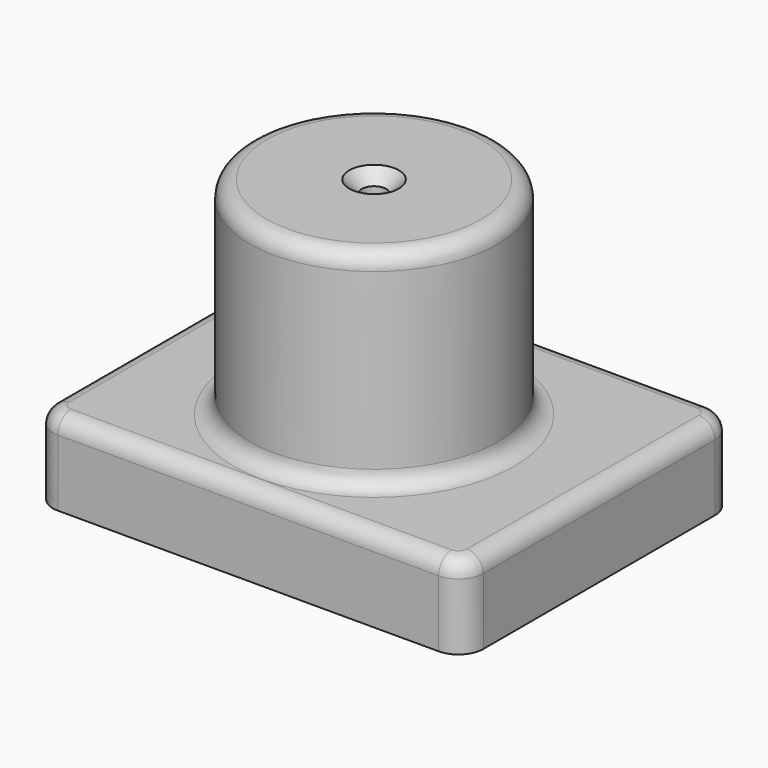
from build123d import *

# Parameters (mm, degrees)
F0_W            = 52
F0_H            = 41
F1_DEPTH        = 10
F3_DEPTH        = 20
F4_R            = 11
F5_DEPTH        = 10.001
F6_R            = 15
F7_DEPTH        = 5
F9_R            = 3
F10_R           = 11.5
F10_R_2         = 9.5
F11_DEPTH       = 35
F12_T3_DEPTH    = 35
F12_T5_DEPTH    = 46
F12_T8_ANGLE    = 90
F12_T10_ANGLE   = 90
F12_T12_ANGLE   = 90
F12_T14_ANGLE   = 90
F13_R           = 10
F14_DEPTH       = 32
F15_R           = 11.5
F16_DEPTH       = 32
F18_D           = 3
F18_CSINK_D     = 6
F18_CSINK_ANGLE = 90


# Not quite as in the source:
# - a fillet or chamfer that OpenCascade refuses, or shapes differently, is made with other operations: its cross-section is extruded or revolved along the edge and cut away or added


with BuildPart() as f1:
    # F0 (on Top) → F1 (new body)
    with BuildSketch(Plane.XY):
        with Locations((26, 20.5)):
            Rectangle(F0_W, F0_H)
    extrude(amount=F1_DEPTH)

    # F2 (on face) → F3 (join)
    with BuildSketch(Plane.XY.offset(10)):
        with BuildLine():
            ThreePointArc((41, 19), (15.3933982822, 29.6066017178), (26, 4))
            ThreePointArc((26, 4), (36.6066017178, 8.3933982822), (41, 19))
        make_face()
        with BuildLine():
            ThreePointArc((37, 19), (33.7781745931, 11.2218254069), (26, 8))
            ThreePointArc((26, 8), (18.2218254069, 26.7781745931), (37, 19))
        make_face(mode=Mode.SUBTRACT)
    extrude(amount=F3_DEPTH)

    # F4 (on face) → F5 (cut, through all)
    with BuildSketch(Plane.XY.offset(10)):
        with Locations((26, 19)):
            Circle(F4_R)
    extrude(amount=-F5_DEPTH, mode=Mode.SUBTRACT)

    # F6 (on face) → F7 (join)
    with BuildSketch(Plane.XY.offset(30)):
        with Locations((26, 19)):
            Circle(F6_R)
    extrude(amount=F7_DEPTH)

    # F8: fillet of radius 2 on 1 edges, made by hand

    # F8_s1 → F8_t2 (revolve, cut)
    with BuildSketch(Plane.XZ.offset(-19)):
        with BuildLine():
            ThreePointArc((41, 33), (40.4142135624, 34.4142135624), (39, 35))
            Line((39, 35), (41, 35))
            Line((41, 35), (41, 33))
        make_face()
    revolve(axis=Axis((26, 19, 35), (0, 0, 1)), mode=Mode.SUBTRACT)

    # F9
    f9_edges = [f1.edges().sort_by_distance(p)[0] for p in [
        (52, 0, 5),
        (0, 0, 5),
        (0, 41, 5),
        (52, 41, 5),
    ]]
    fillet(f9_edges, radius=F9_R)

    # F10 (on face) → F11 (join)
    with BuildSketch(Plane(origin=(0, 0, 0), x_dir=(1, 0, 0), z_dir=(0, 0, -1))):
        with Locations((26, -19)):
            Circle(F10_R)
        with Locations((26, -19)):
            Circle(F10_R_2, mode=Mode.SUBTRACT)
    extrude(amount=-F11_DEPTH)

    # F12: fillet of radius 2 on 9 edges, made by hand

    # F12_s1 → F12_t2 (revolve)
    with BuildSketch(Plane.YZ.offset(26)):
        with BuildLine():
            ThreePointArc((1.9990343146, 9.9996), (3.4142135624, 10.5857864376), (4.0004, 12.0009656854))
            Line((4.0004, 12.0009656854), (4.2005365685, 12.0009656854))
            ThreePointArc((4.2005365685, 12.0009656854), (4.2001365685, 11.0004828427), (4.2001365685, 10))
            Line((4.2001365685, 10), (4, 9.7998634315))
            ThreePointArc((4, 9.7998634315), (2.9995171573, 9.7998634315), (1.9990343146, 9.7994634315))
            Line((1.9990343146, 9.7994634315), (1.9990343146, 9.9996))
        make_face()
    revolve(axis=Axis((26, 19, 10), (0, 0, 1)))

    # F12_s4 → F12_t3 (cut)
    with BuildSketch(Plane.XZ.offset(-38)):
        with BuildLine():
            ThreePointArc((-0.0004, 7.9990343146), (0.5857864376, 9.4142135624), (2.0009656854, 10.0004))
            Line((2.0009656854, 10.0004), (2.0009656854, 10.2005365685))
            ThreePointArc((2.0009656854, 10.2005365685), (1.0004828427, 10.2001365685), (0, 10.2001365685))
            Line((0, 10.2001365685), (-0.2001365685, 10))
            ThreePointArc((-0.2001365685, 10), (-0.2001365685, 8.9995171573), (-0.2005365685, 7.9990343146))
            Line((-0.2005365685, 7.9990343146), (-0.0004, 7.9990343146))
        make_face()
        with BuildLine():
            ThreePointArc((49.9990343146, 10.0004), (51.4142135624, 9.4142135624), (52.0004, 7.9990343146))
            Line((52.0004, 7.9990343146), (52.2005365685, 7.9990343146))
            ThreePointArc((52.2005365685, 7.9990343146), (52.2001365685, 8.9995171573), (52.2001365685, 10))
            Line((52.2001365685, 10), (52, 10.2001365685))
            ThreePointArc((52, 10.2001365685), (50.9995171573, 10.2001365685), (49.9990343146, 10.2005365685))
            Line((49.9990343146, 10.2005365685), (49.9990343146, 10.0004))
        make_face()
    extrude(amount=F12_T3_DEPTH, mode=Mode.SUBTRACT)

    # F12_s6 → F12_t5 (cut)
    with BuildSketch(Plane.YZ.offset(3)):
        with BuildLine():
            ThreePointArc((38.9990343146, 10.0004), (40.4142135624, 9.4142135624), (41.0004, 7.9990343146))
            Line((41.0004, 7.9990343146), (41.2005365685, 7.9990343146))
            ThreePointArc((41.2005365685, 7.9990343146), (41.2001365685, 8.9995171573), (41.2001365685, 10))
            Line((41.2001365685, 10), (41, 10.2001365685))
            ThreePointArc((41, 10.2001365685), (39.9995171573, 10.2001365685), (38.9990343146, 10.2005365685))
            Line((38.9990343146, 10.2005365685), (38.9990343146, 10.0004))
        make_face()
        with BuildLine():
            ThreePointArc((2.0009656854, 10.0004), (0.5857864376, 9.4142135624), (-0.0004, 7.9990343146))
            Line((-0.0004, 7.9990343146), (-0.2005365685, 7.9990343146))
            ThreePointArc((-0.2005365685, 7.9990343146), (-0.2001365685, 8.9995171573), (-0.2001365685, 10))
            Line((-0.2001365685, 10), (0, 10.2001365685))
            ThreePointArc((0, 10.2001365685), (1.0004828427, 10.2001365685), (2.0009656854, 10.2005365685))
            Line((2.0009656854, 10.2005365685), (2.0009656854, 10.0004))
        make_face()
    extrude(amount=F12_T5_DEPTH, mode=Mode.SUBTRACT)

    # F12_s7 → F12_t8 (revolve, cut)
    with BuildSketch(Plane.XZ.offset(-38)):
        with BuildLine():
            ThreePointArc((2.0009656854, 10.0004), (0.5857864376, 9.4142135624), (-0.0004, 7.9990343146))
            Line((-0.0004, 7.9990343146), (-0.2005365685, 7.9990343146))
            ThreePointArc((-0.2005365685, 7.9990343146), (-0.2001365685, 8.9995171573), (-0.2001365685, 10))
            Line((-0.2001365685, 10), (0, 10.2001365685))
            ThreePointArc((0, 10.2001365685), (1.0004828427, 10.2001365685), (2.0009656854, 10.2005365685))
            Line((2.0009656854, 10.2005365685), (2.0009656854, 10.0004))
        make_face()
    revolve(axis=Axis((3, 38, 10), (0, 0, -1)), revolution_arc=F12_T8_ANGLE, mode=Mode.SUBTRACT)

    # F12_s9 → F12_t10 (revolve, cut)
    with BuildSketch(Plane.XZ.offset(-3)):
        with BuildLine():
            ThreePointArc((2.0009656854, 10.0004), (0.5857864376, 9.4142135624), (-0.0004, 7.9990343146))
            Line((-0.0004, 7.9990343146), (-0.2005365685, 7.9990343146))
            ThreePointArc((-0.2005365685, 7.9990343146), (-0.2001365685, 8.9995171573), (-0.2001365685, 10))
            Line((-0.2001365685, 10), (0, 10.2001365685))
            ThreePointArc((0, 10.2001365685), (1.0004828427, 10.2001365685), (2.0009656854, 10.2005365685))
            Line((2.0009656854, 10.2005365685), (2.0009656854, 10.0004))
        make_face()
    revolve(axis=Axis((3, 3, 10), (0, 0, 1)), revolution_arc=F12_T10_ANGLE, mode=Mode.SUBTRACT)

    # F12_s11 → F12_t12 (revolve, cut)
    with BuildSketch(Plane.YZ.offset(49)):
        with BuildLine():
            ThreePointArc((38.9990343146, 10.0004), (40.4142135624, 9.4142135624), (41.0004, 7.9990343146))
            Line((41.0004, 7.9990343146), (41.2005365685, 7.9990343146))
            ThreePointArc((41.2005365685, 7.9990343146), (41.2001365685, 8.9995171573), (41.2001365685, 10))
            Line((41.2001365685, 10), (41, 10.2001365685))
            ThreePointArc((41, 10.2001365685), (39.9995171573, 10.2001365685), (38.9990343146, 10.2005365685))
            Line((38.9990343146, 10.2005365685), (38.9990343146, 10.0004))
        make_face()
    revolve(axis=Axis((49, 38, 10), (0, 0, -1)), revolution_arc=F12_T12_ANGLE, mode=Mode.SUBTRACT)

    # F12_s13 → F12_t14 (revolve, cut)
    with BuildSketch(Plane.YZ.offset(49)):
        with BuildLine():
            ThreePointArc((2.0009656854, 10.0004), (0.5857864376, 9.4142135624), (-0.0004, 7.9990343146))
            Line((-0.0004, 7.9990343146), (-0.2005365685, 7.9990343146))
            ThreePointArc((-0.2005365685, 7.9990343146), (-0.2001365685, 8.9995171573), (-0.2001365685, 10))
            Line((-0.2001365685, 10), (0, 10.2001365685))
            ThreePointArc((0, 10.2001365685), (1.0004828427, 10.2001365685), (2.0009656854, 10.2005365685))
            Line((2.0009656854, 10.2005365685), (2.0009656854, 10.0004))
        make_face()
    revolve(axis=Axis((49, 3, 10), (0, 0, 1)), revolution_arc=F12_T14_ANGLE, mode=Mode.SUBTRACT)

    # F13 (on face) → F14 (cut)
    with BuildSketch(Plane(origin=(0, 0, 0), x_dir=(1, 0, 0), z_dir=(0, 0, -1))):
        with Locations((26, -19)):
            Circle(F13_R)
    extrude(amount=-F14_DEPTH, mode=Mode.SUBTRACT)

    # F15 (on face) → F16 (cut, through all)
    with BuildSketch(Plane(origin=(0, 0, 0), x_dir=(1, 0, 0), z_dir=(0, 0, -1))):
        with Locations((26, -19)):
            Circle(F15_R)
    extrude(amount=-F16_DEPTH, mode=Mode.SUBTRACT)

    # F18 (through all)
    with Locations(Plane.XY.offset(35)):
        with Locations((26, 19)):
            CounterSinkHole(F18_D / 2, F18_CSINK_D / 2, counter_sink_angle=F18_CSINK_ANGLE)


solid = f1.part
